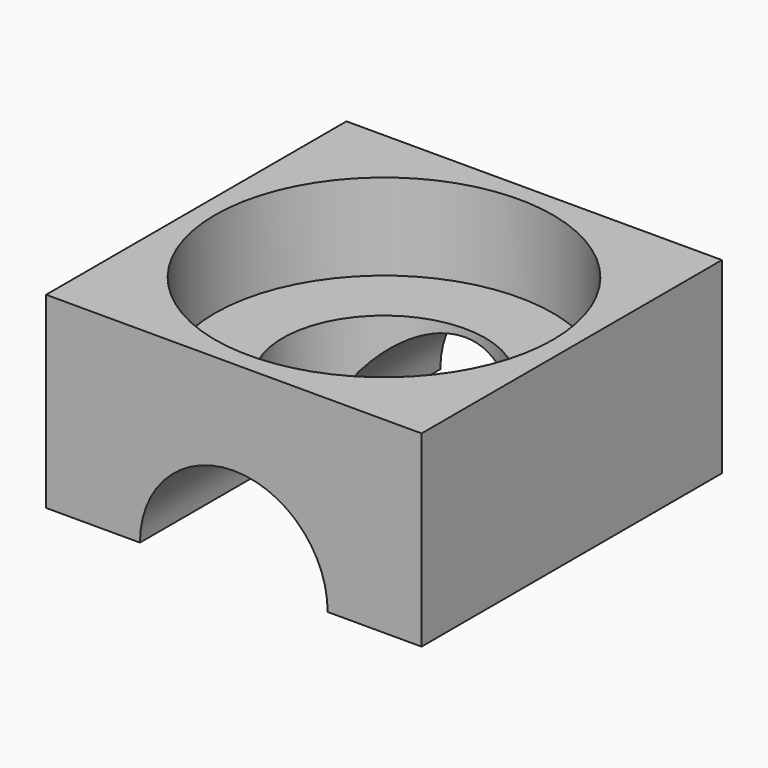
from build123d import *

# Parameters (mm, degrees)
F1_DEPTH = 50
F2_R     = 27
F3_DEPTH = 50
F4_R     = 45
F5_DEPTH = 23


with BuildPart() as f1:
    # F0 (on Front) → F1 (new body, symmetric)
    with BuildSketch(Plane.XZ):
        with BuildLine():
            ThreePointArc((0, 25), (17.67767, 17.67767), (25, 0))
            Line((25, 0), (50, 0))
            Line((50, 0), (50, 50))
            Line((50, 50), (-50, 50))
            Line((-50, 50), (-50, 0))
            Line((-50, 0), (-25, 0))
            ThreePointArc((-25, 0), (-17.67767, 17.67767), (0, 25))
        make_face()
    extrude(amount=F1_DEPTH, both=True)

    # F2 (on face) → F3 (cut)
    with BuildSketch(Plane.XY.offset(50)):
        Circle(F2_R)
    extrude(amount=-F3_DEPTH, mode=Mode.SUBTRACT)

    # F4 (on face) → F5 (cut)
    with BuildSketch(Plane.XY.offset(50)):
        Circle(F4_R)
    extrude(amount=-F5_DEPTH, mode=Mode.SUBTRACT)


solid = f1.part
